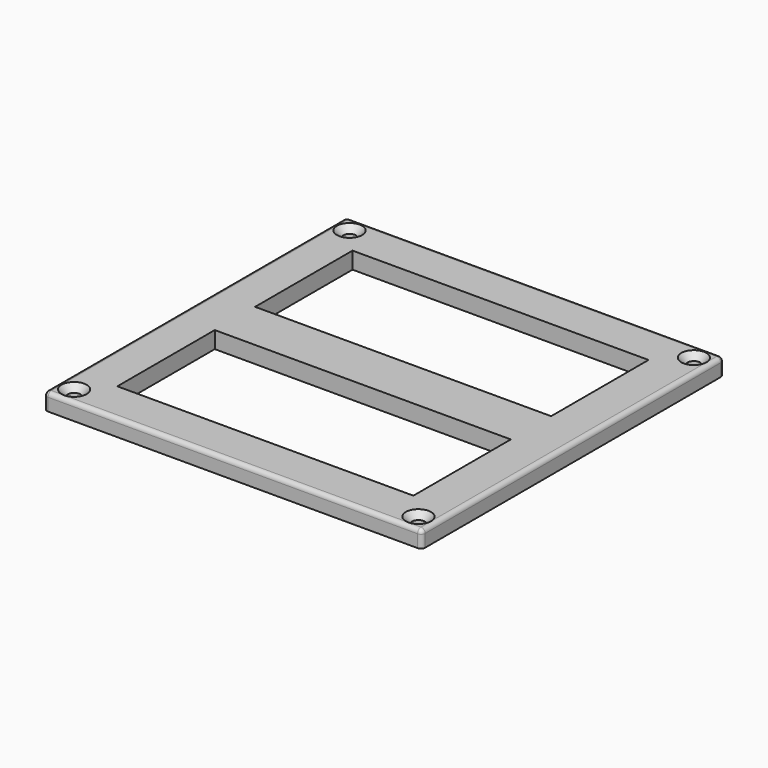
from build123d import *

# Parameters (mm, degrees)
F0_W           = 90
F0_H           = 90
F0_W_2         = 70.5104
F0_H_2         = 29.0068
F0_W_3         = 70.5
F0_H_3         = 29
F1_DEPTH       = 4
F3_D           = 3
F3_CSINK_D     = 6
F3_CSINK_ANGLE = 90
F4_T1_DEPTH    = 88
F4_T3_DEPTH    = 88
F4_T5_DEPTH    = 5.5
F4_S9_W        = 1
F4_S9_H        = 1
F4_T10_DEPTH   = 1
F4_S15_W       = 1
F4_S15_H       = 1
F4_T16_DEPTH   = 1
F4_S21_W       = 1
F4_S21_H       = 1
F4_T22_DEPTH   = 1
F4_S27_W       = 1
F4_S27_H       = 1
F4_T28_DEPTH   = 1


# Not quite as in the source:
# - a fillet or chamfer that OpenCascade refuses, or shapes differently, is made with other operations: its cross-section is extruded or revolved along the edge and cut away or added


with BuildPart() as f1:
    # F0 (on Top) → F1 (new body)
    with BuildSketch(Plane.XY):
        Rectangle(F0_W, F0_H)
        with Locations((-0.2552, -20.4966)):
            Rectangle(F0_W_2, F0_H_2, mode=Mode.SUBTRACT)
        with Locations((-0.25, 20.5)):
            Rectangle(F0_W_3, F0_H_3, mode=Mode.SUBTRACT)
    extrude(amount=F1_DEPTH)

    # F3 (through all)
    with Locations(Plane.XY.offset(4)):
        with Locations((-41, 41), (41, 41), (41, -41), (-41, -41)):
            CounterSinkHole(F3_D / 2, F3_CSINK_D / 2, counter_sink_angle=F3_CSINK_ANGLE)

    # F4: fillet of radius 1 on 8 edges, made by hand

    # F4_s2 → F4_t1 (cut)
    with BuildSketch(Plane.YZ.offset(-44)):
        with BuildLine():
            ThreePointArc((45, 3), (44.7071067812, 3.7071067812), (44, 4))
            Line((44, 4), (45, 4))
            Line((45, 4), (45, 3))
        make_face()
        with BuildLine():
            ThreePointArc((-44, 4), (-44.7071067812, 3.7071067812), (-45, 3))
            Line((-45, 3), (-45, 4))
            Line((-45, 4), (-44, 4))
        make_face()
    extrude(amount=F4_T1_DEPTH, mode=Mode.SUBTRACT)

    # F4_s4 → F4_t3 (cut)
    with BuildSketch(Plane.XZ.offset(-44)):
        with BuildLine():
            ThreePointArc((-45, 3), (-44.7071067812, 3.7071067812), (-44, 4))
            Line((-44, 4), (-45, 4))
            Line((-45, 4), (-45, 3))
        make_face()
        with BuildLine():
            ThreePointArc((45, 3), (44.7071067812, 3.7071067812), (44, 4))
            Line((44, 4), (45, 4))
            Line((45, 4), (45, 3))
        make_face()
    extrude(amount=F4_T3_DEPTH, mode=Mode.SUBTRACT)

    # F4_s6 → F4_t5 (cut)
    with BuildSketch(Plane.XY.offset(-2.5)):
        with BuildLine():
            ThreePointArc((45, -44), (44.7071067812, -44.7071067812), (44, -45))
            Line((44, -45), (45, -45))
            Line((45, -45), (45, -44))
        make_face()
        with BuildLine():
            ThreePointArc((44, 45), (44.7071067812, 44.7071067812), (45, 44))
            Line((45, 44), (45, 45))
            Line((45, 45), (44, 45))
        make_face()
        with BuildLine():
            ThreePointArc((-44, 45), (-44.7071067812, 44.7071067812), (-45, 44))
            Line((-45, 44), (-45, 45))
            Line((-45, 45), (-44, 45))
        make_face()
        with BuildLine():
            ThreePointArc((-45, -44), (-44.7071067812, -44.7071067812), (-44, -45))
            Line((-44, -45), (-45, -45))
            Line((-45, -45), (-45, -44))
        make_face()
    extrude(amount=F4_T5_DEPTH, mode=Mode.SUBTRACT)


with BuildPart() as f4_tool8:
    # F4_s9 → F4_t10 (new body)
    with BuildSketch(Plane.XZ.offset(-44)):
        with Locations((44.5, 3.5)):
            Rectangle(F4_S9_W, F4_S9_H)
    extrude(amount=-F4_T10_DEPTH)

    # F4_s11 → F4_t12 (revolve, cut)
    with BuildSketch(Plane(origin=(44, 44, 3), x_dir=(-0.7071067812, 0, -0.7071067812), z_dir=(0.7071067812, 0, -0.7071067812))):
        with BuildLine():
            ThreePointArc((0, -1), (1, 0), (0, 1))
            Line((0, 1), (0, -1))
        make_face()
    revolve(axis=Axis((44, 44, 3), (0, 1, 0)), mode=Mode.SUBTRACT)


with BuildPart() as f1_1:
    add(f1.part)

    # F4_t7: cut F4_tool8
    add(f4_tool8.part, mode=Mode.SUBTRACT)


with BuildPart() as f4_tool14:
    # F4_s15 → F4_t16 (new body)
    with BuildSketch(Plane.XZ.offset(-44)):
        with Locations((-44.5, 3.5)):
            Rectangle(F4_S15_W, F4_S15_H)
    extrude(amount=-F4_T16_DEPTH)

    # F4_s17 → F4_t18 (revolve, cut)
    with BuildSketch(Plane(origin=(-44, 44, 3), x_dir=(0.7071067812, 0, -0.7071067812), z_dir=(0.7071067812, 0, 0.7071067812))):
        with BuildLine():
            ThreePointArc((0, -1), (1, 0), (0, 1))
            Line((0, 1), (0, -1))
        make_face()
    revolve(axis=Axis((-44, 44, 3), (0, 1, 0)), mode=Mode.SUBTRACT)


with BuildPart() as f1_2:
    add(f1_1.part)

    # F4_t13: cut F4_tool14
    add(f4_tool14.part, mode=Mode.SUBTRACT)


with BuildPart() as f4_tool20:
    # F4_s21 → F4_t22 (new body)
    with BuildSketch(Plane.YZ.offset(-44)):
        with Locations((-44.5, 3.5)):
            Rectangle(F4_S21_W, F4_S21_H)
    extrude(amount=-F4_T22_DEPTH)

    # F4_s23 → F4_t24 (revolve, cut)
    with BuildSketch(Plane(origin=(-44, -44, 3), x_dir=(0, 0.7071067812, -0.7071067812), z_dir=(0, 0.7071067812, 0.7071067812))):
        with BuildLine():
            ThreePointArc((0, -1), (1, 0), (0, 1))
            Line((0, 1), (0, -1))
        make_face()
    revolve(axis=Axis((-44, -44, 3), (-1, 0, 0)), mode=Mode.SUBTRACT)


with BuildPart() as f1_3:
    add(f1_2.part)

    # F4_t19: cut F4_tool20
    add(f4_tool20.part, mode=Mode.SUBTRACT)


with BuildPart() as f4_tool26:
    # F4_s27 → F4_t28 (new body)
    with BuildSketch(Plane.YZ.offset(44)):
        with Locations((-44.5, 3.5)):
            Rectangle(F4_S27_W, F4_S27_H)
    extrude(amount=F4_T28_DEPTH)

    # F4_s29 → F4_t30 (revolve, cut)
    with BuildSketch(Plane(origin=(44, -44, 3), x_dir=(0, 0.7071067812, -0.7071067812), z_dir=(0, -0.7071067812, -0.7071067812))):
        with BuildLine():
            ThreePointArc((0, -1), (1, 0), (0, 1))
            Line((0, 1), (0, -1))
        make_face()
    revolve(axis=Axis((44, -44, 3), (1, 0, 0)), mode=Mode.SUBTRACT)


with BuildPart() as f1_4:
    add(f1_3.part)

    # F4_t25: cut F4_tool26
    add(f4_tool26.part, mode=Mode.SUBTRACT)


solid = f1_4.part
